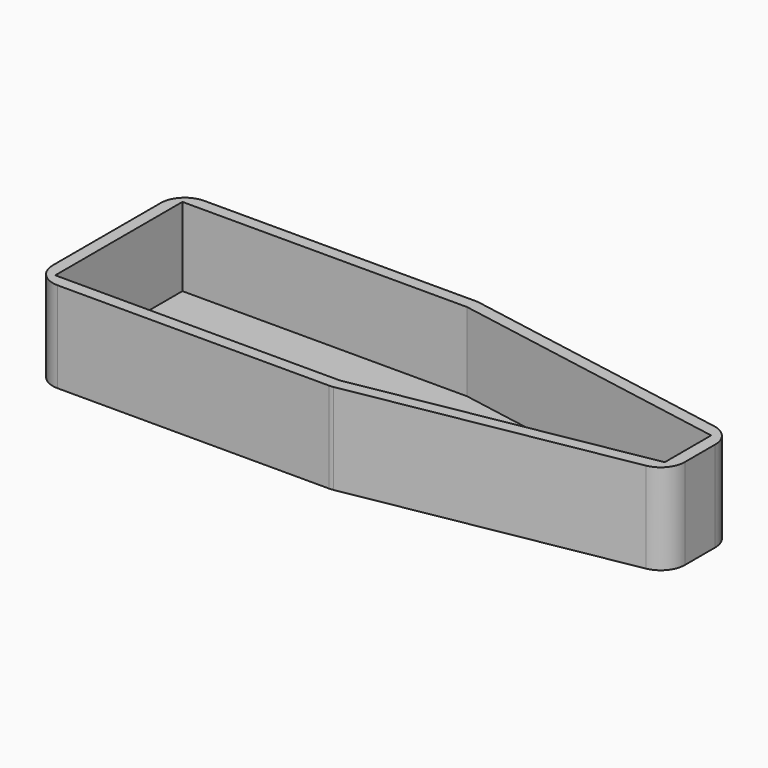
from build123d import *

# Parameters (mm, degrees)
F1_DEPTH    = 8.255
F2_T        = 2.54
F3_T1_DEPTH = 40.3429500211
F3_T3_DEPTH = 21.284150325
F3_T5_DEPTH = 44.45


# Not quite as in the source:
# - a fillet or chamfer that OpenCascade refuses, or shapes differently, is made with other operations: its cross-section is extruded or revolved along the edge and cut away or added


with BuildPart() as f1:
    # F0 (on Top) → F1 (new body, symmetric)
    with BuildSketch(Plane.XY):
        Polygon((0, 16.7005), (-59.7916, 16.7005), (-59.7916, -16.7005), (0, -16.7005), (59.7916, -6.1001079157), (59.7916, 6.1001079157), align=None)
    extrude(amount=F1_DEPTH, both=True)

    # F2
    f2_openings = [f1.faces().sort_by_distance(p)[0] for p in [
        (-7.518342, 0, 8.255),
    ]]
    offset(amount=F2_T, openings=f2_openings, kind=Kind.INTERSECTION)

    # F3: fillet of radius 5.08 on 6 edges, made by hand

    # F3_s2 → F3_t1 (cut)
    with BuildSketch(Plane.XY.offset(-21.4414750105)):
        with BuildLine():
            ThreePointArc((58.1383992054, 8.9728112312), (61.1446283818, 7.2343585343), (62.3316, 3.9708129136))
            Line((62.3316, 3.9708129136), (62.3316, 8.2294029178))
            Line((62.3316, 8.2294029178), (58.1383992054, 8.9728112312))
        make_face()
        with BuildLine():
            ThreePointArc((62.3316, -3.9708129136), (61.1446283818, -7.2343585343), (58.1383992054, -8.9728112312))
            Line((58.1383992054, -8.9728112312), (62.3316, -8.2294029178))
            Line((62.3316, -8.2294029178), (62.3316, -3.9708129136))
        make_face()
    extrude(amount=F3_T1_DEPTH, mode=Mode.SUBTRACT)

    # F3_s4 → F3_t3 (cut)
    with BuildSketch(Plane.XY.offset(-11.9120751625)):
        with BuildLine():
            ThreePointArc((0.6633841729, 19.1624983176), (0.2216964966, 19.2209620072), (-0.2234150325, 19.2405))
            Line((-0.2234150325, 19.2405), (0.2234150325, 19.2405))
            Line((0.2234150325, 19.2405), (0.6633841729, 19.1624983176))
        make_face()
        with BuildLine():
            ThreePointArc((0.6633841729, -19.1624983176), (0.2216964966, -19.2209620072), (-0.2234150325, -19.2405))
            Line((-0.2234150325, -19.2405), (0.2234150325, -19.2405))
            Line((0.2234150325, -19.2405), (0.6633841729, -19.1624983176))
        make_face()
    extrude(amount=F3_T3_DEPTH, mode=Mode.SUBTRACT)

    # F3_s6 → F3_t5 (cut)
    with BuildSketch(Plane.XY.offset(-23.495)):
        with BuildLine():
            ThreePointArc((-57.2516, -19.2405), (-60.8437024484, -17.7526024484), (-62.3316, -14.1605))
            Line((-62.3316, -14.1605), (-62.3316, -19.2405))
            Line((-62.3316, -19.2405), (-57.2516, -19.2405))
        make_face()
        with BuildLine():
            ThreePointArc((-62.3316, 14.1605), (-60.8437024484, 17.7526024484), (-57.2516, 19.2405))
            Line((-57.2516, 19.2405), (-62.3316, 19.2405))
            Line((-62.3316, 19.2405), (-62.3316, 14.1605))
        make_face()
    extrude(amount=F3_T5_DEPTH, mode=Mode.SUBTRACT)


solid = f1.part
